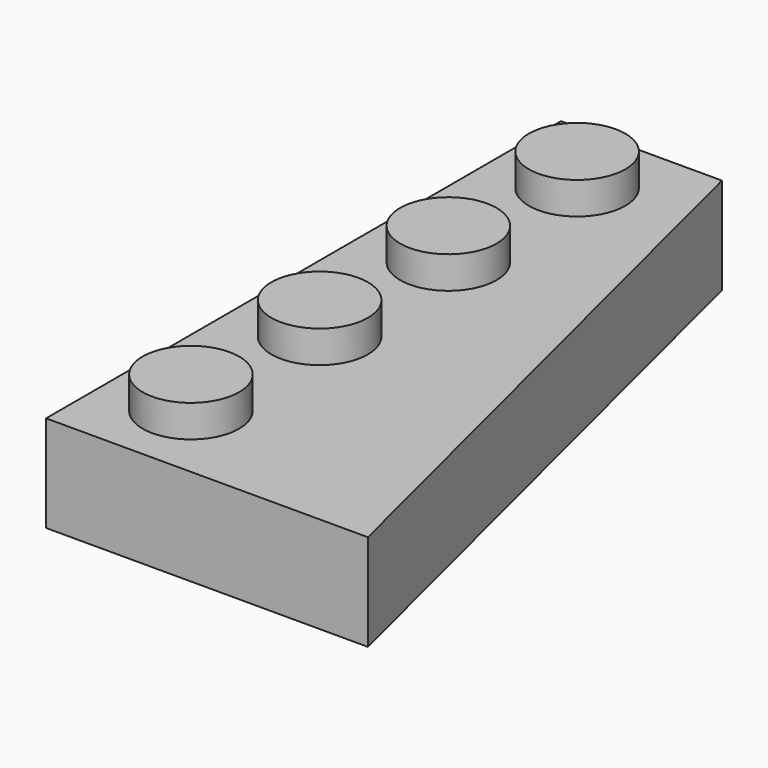
from build123d import *

# Parameters (mm, degrees)
F0_R     = 2.38125
F1_DEPTH = 3.175
F2_DEPTH = 4.7625
F3_T     = -1.5875
F4_R     = 3.175
F4_R_2   = 2.38125
F5_DEPTH = 1.5875


with BuildPart() as f1:
    # F0 (on Top) → F1 (new body)
    with BuildSketch(Plane.XY):
        Polygon((0, 15.875), (-7.9375, 15.875), (-7.9375, -15.875), (7.9375, -15.875), align=None)
        with Locations((-3.96875, -11.90625)):
            Circle(F0_R, mode=Mode.SUBTRACT)
        with Locations((-3.96875, -3.96875)):
            Circle(F0_R, mode=Mode.SUBTRACT)
        with Locations((-3.96875, 3.96875)):
            Circle(F0_R, mode=Mode.SUBTRACT)
        with Locations((-3.96875, 11.90625)):
            Circle(F0_R, mode=Mode.SUBTRACT)
    extrude(amount=F1_DEPTH)

    # F0 (on Top) → F2 (join)
    with BuildSketch(Plane.XY):
        with Locations((-3.96875, 11.90625)):
            Circle(F0_R)
        with Locations((-3.96875, 3.96875)):
            Circle(F0_R)
        with Locations((-3.96875, -3.96875)):
            Circle(F0_R)
        with Locations((-3.96875, -11.90625)):
            Circle(F0_R)
    extrude(amount=F2_DEPTH)

    # F3
    f3_openings = [f1.faces().sort_by_distance(p)[0] for p in [
        (-1.763889, -1.763889, 0),
    ]]
    offset(amount=F3_T, openings=f3_openings, kind=Kind.INTERSECTION)

    # F2_face (on face) + F4 (on face) → F5 (join)
    with BuildSketch(Plane(origin=(-1.7638745265, -1.3908157983, 0), x_dir=(1, 0, 0), z_dir=(0, 0, -1))):
        Polygon((-6.1736254735, -17.2658157983), (1.7638745265, -17.2658157983), (9.7013745265, 14.4841842017), (-6.1736254735, 14.4841842017), align=None)
        Polygon((0.5243919814, -15.6783157983), (-4.5861254735, -15.6783157983), (-4.5861254735, 12.8966842017), (7.6681419814, 12.8966842017), align=None, mode=Mode.SUBTRACT)
    with BuildSketch(Plane(origin=(0, 0, 1.5875), x_dir=(1, 0, 0), z_dir=(0, 0, -1))):
        with BuildLine():
            Line((0.8992491716, -5.7325731328), (1.0932302062, -4.9566489946))
            ThreePointArc((1.0932302062, -4.9566489946), (-3.080202438, -7.1674493905), (-0.4381385265, -11.0821239253))
            Line((-0.4381385265, -11.0821239253), (-0.244157492, -10.3061997871))
            ThreePointArc((-0.244157492, -10.3061997871), (-2.3101518285, -7.3599620429), (0.8992491716, -5.7325731328))
        make_face()
        with BuildLine():
            ThreePointArc((2.7353766172, 1.6119366495), (-3.080202438, 0.7700506095), (1.6550091801, -2.7095330988))
            Line((1.6550091801, -2.7095330988), (2.0152745824, -1.2684714896))
            ThreePointArc((2.0152745824, -1.2684714896), (-2.3101518285, 0.5775379571), (2.3751112149, 0.1708750402))
            Line((2.3751112149, 0.1708750402), (2.7353766172, 1.6119366495))
        make_face()
        with Locations((0, 7.9375)):
            Circle(F4_R)
        with Locations((0, 7.9375)):
            Circle(F4_R_2, mode=Mode.SUBTRACT)
    extrude(amount=F5_DEPTH)


solid = f1.part
